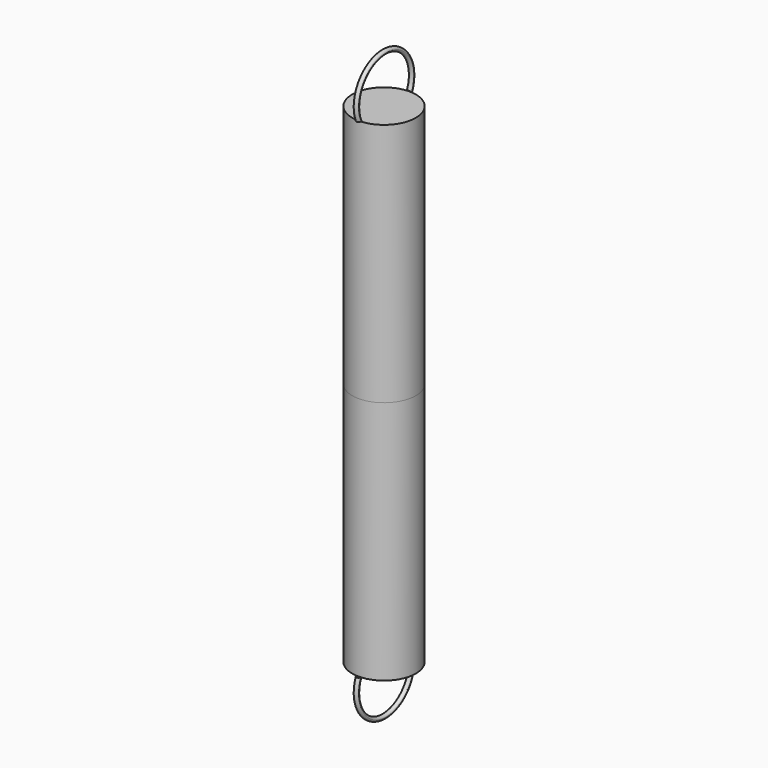
from build123d import *

# Parameters (mm, degrees)
F0_R     = 3.57
F1_DEPTH = 27.5


# Not quite as in the source:
# - the program builds the solid bodies; features that only make, move or delete a surface that nothing else refers to are left out


with BuildPart() as f1:
    # F0 (on Top) → F1 (new body)
    with BuildSketch(Plane.XY):
        Circle(F0_R)
    extrude(amount=F1_DEPTH)


with BuildPart() as f4:
    # F4: sweep along a path in F2
    with BuildLine(Plane.YZ) as f4_path:
        ThreePointArc((3.57, 27.5), (0, 32.8723248831), (-3.57, 27.5))
    # F3 (on face) → F4 (sweep)
    with BuildSketch(Plane.XY.offset(27.5)):
        with BuildLine():
            ThreePointArc((-0.2498467054, -3.5612464986), (-0.0043774218, -3.8199616734), (0.25, -3.57))
            ThreePointArc((0.25, -3.57), (0.2499616734, -3.5656225782), (0.2498467054, -3.5612464986))
            ThreePointArc((0.2498467054, -3.5612464986), (0, -3.57), (-0.2498467054, -3.5612464986))
        make_face()
        with BuildLine():
            ThreePointArc((-0.2498467054, -3.5612464986), (0, -3.57), (0.2498467054, -3.5612464986))
            ThreePointArc((0.2498467054, -3.5612464986), (0, -3.32), (-0.2498467054, -3.5612464986))
        make_face()
    sweep(path=f4_path.line)


with BuildPart() as f5_1:
    # F5: instance of F4
    add(f4.part.mirror(Plane.XY))


with BuildPart() as f5_2:
    # F5: instance of F1
    add(f1.part.mirror(Plane.XY))


solid = Compound([f1.part, f4.part, f5_1.part, f5_2.part])
